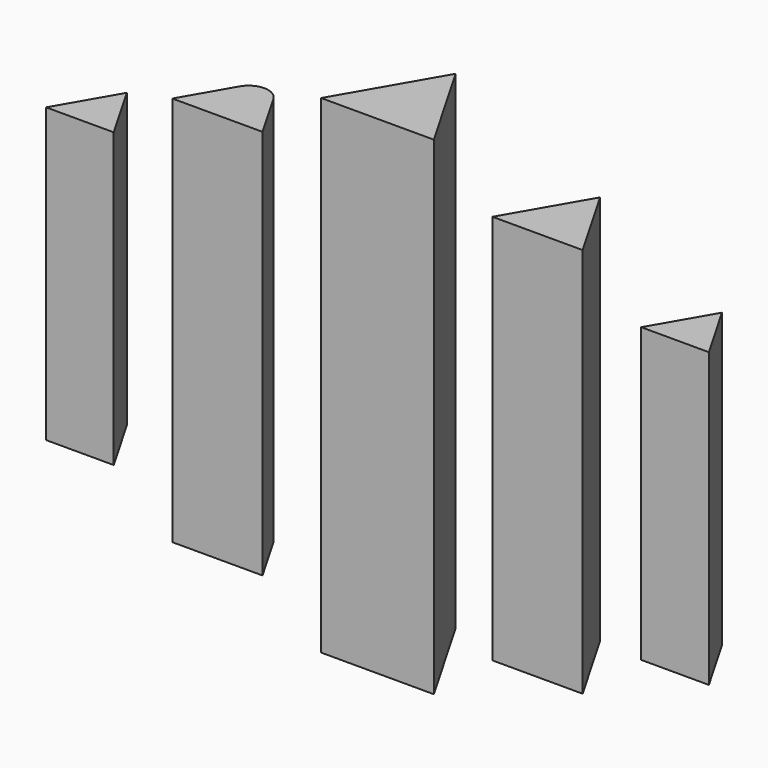
from build123d import *

# Parameters (mm, degrees)
F1_DEPTH = 12.5
F2_DEPTH = 10
F3_DEPTH = 7.5
F7_R     = 1


# Not quite as in the source:
# - the program builds the solid bodies; features that only make, move or delete a surface that nothing else refers to are left out


with BuildPart() as f1:
    # F0 (on Top) → F1 (new body, symmetric)
    with BuildSketch(Plane.XY):
        Polygon((-2.8867513459, 0), (2.8867513459, 0), (0, 5), align=None)
    extrude(amount=F1_DEPTH, both=True)


with BuildPart() as f2:
    # F0 (on Top) → F2 (new body, symmetric)
    with BuildSketch(Plane.XY):
        Polygon((-10.5055534995, 0), (-5.8867513459, 0), (-8.1961524227, 4), align=None)
    extrude(amount=F2_DEPTH, both=True)


with BuildPart() as f3:
    # F0 (on Top) → F3 (new body, symmetric)
    with BuildSketch(Plane.XY):
        Polygon((-16.9696551146, 0), (-13.5055534995, 0), (-15.237604307, 3), align=None)
    extrude(amount=F3_DEPTH, both=True)


with BuildPart() as f4_1:
    # F4: instance of F2
    add(f2.part.mirror(Plane.YZ))


with BuildPart() as f4_2:
    # F4: instance of F3
    add(f3.part.mirror(Plane.YZ))


with BuildPart() as f2_1:
    add(f2.part)

    # F7
    f7_edges = [f2_1.edges().sort_by_distance(p)[0] for p in [
        (-8.196152, 4, 0),
    ]]
    fillet(f7_edges, radius=F7_R)


solid = Compound([f1.part, f3.part, f4_1.part, f4_2.part, f2_1.part])
